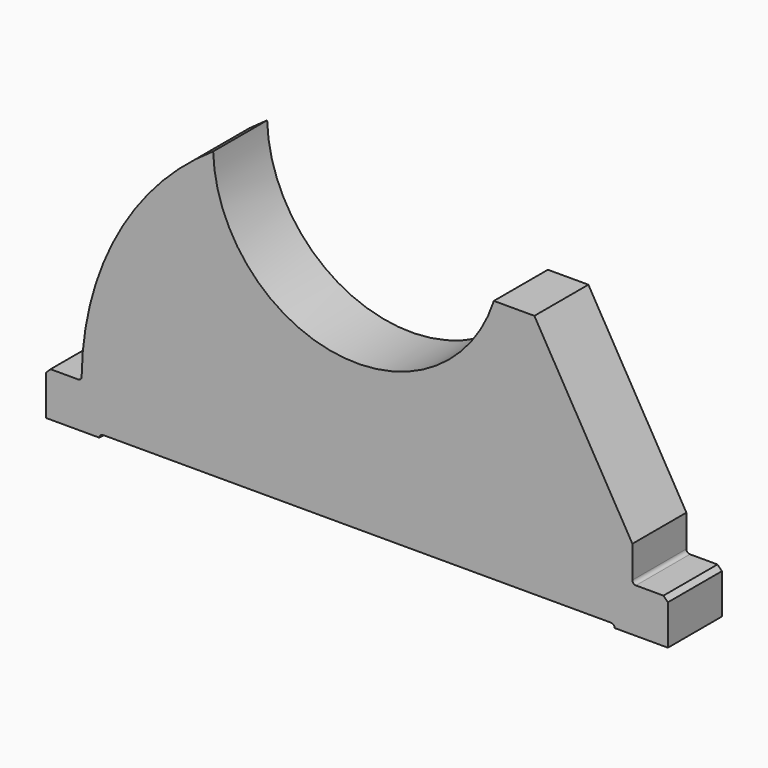
from build123d import *

# Parameters (mm, degrees)
F1_DEPTH = 38


# Not quite as in the source:
# - ends of sketch curves that miss each other by under 0.0002 mm in the source are joined


with BuildPart() as f1:
    # F0 (on Front) → F1 (new body)
    with BuildSketch(Plane.XZ):
        with BuildLine():
            Line((485.006122, -179.853302), (485.006122, -202.353302))
            Line((485.006122, -202.353302), (515.006122, -202.353302))
            ThreePointArc((515.006122, -202.353302), (515.5919084376, -200.9390884376), (517.006122, -200.353302))
            Line((517.006122, -200.353302), (803.006122, -200.353302))
            ThreePointArc((803.006122, -200.353302), (804.4203355624, -200.9390884376), (805.006122, -202.353302))
            Line((805.006122, -202.353302), (835.006122, -202.353302))
            Line((835.006122, -202.353302), (835.006122, -179.853302))
            Line((835.006122, -179.853302), (832.506122, -177.353302))
            Line((832.506122, -177.353302), (817.006122, -177.353302))
            ThreePointArc((817.006122, -177.353302), (815.5919084376, -176.7675155624), (815.006122, -175.353302))
            Line((815.006122, -175.353302), (815.006122, -157.353302))
            Line((815.006122, -157.353302), (759.841906, -62.353302))
            Line((759.841906, -62.353302), (737.051563, -62.353302))
            ThreePointArc((737.051563, -62.353302), (648.507993777, -117.5330565978), (579.0399418017, -39.6937430057))
            ThreePointArc((579.0399418017, -39.6937430057), (525.1590968788, -98.3321699305), (505.0179550476, -175.3772540006))
            ThreePointArc((505.0179550476, -175.3772540006), (504.4238177463, -176.7759586679), (503.018098, -177.353302))
            Line((503.018098, -177.353302), (487.506122, -177.353302))
            Line((487.506122, -177.353302), (485.006122, -179.853302))
        make_face()
    extrude(amount=F1_DEPTH)


solid = f1.part
